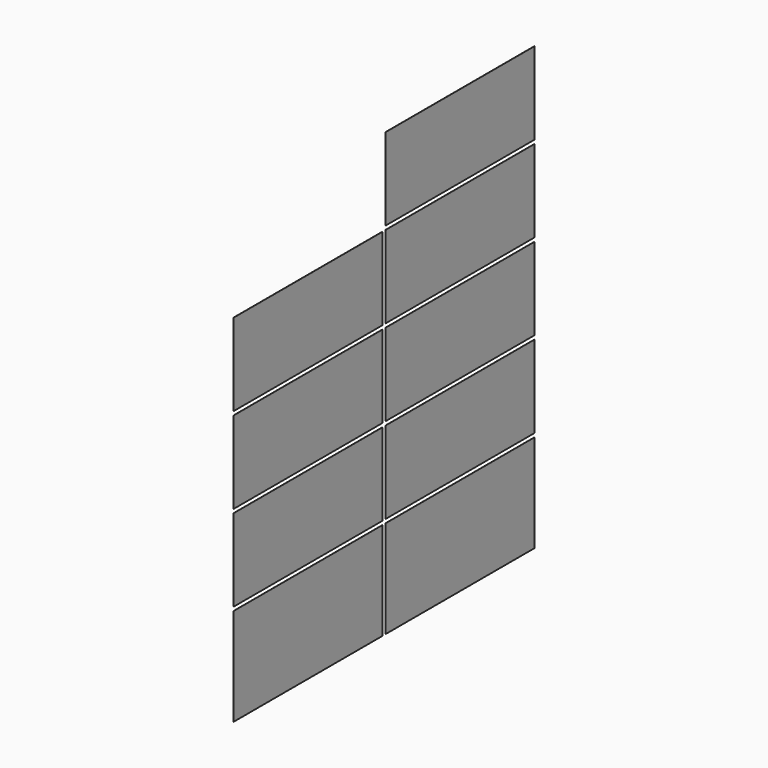
from build123d import *

# Parameters (mm, degrees)
F1_DEPTH = 0.012


# Not quite as in the source:
# - a feature names something its author has since deleted; it is built from what else it names


with BuildPart() as f1:
    # F0 (on Right) → F1 (new body)
    with BuildSketch(Plane.YZ):
        Polygon((50, -12.238), (50, -1.304), (25.25, -1.304), (25.25, -3.119), (25.25, -6.119), (25.25, -6.521), (25.25, -7.021), (25.25, -9.119), (25.25, -12.238), align=None)
    extrude(amount=F1_DEPTH)


with BuildPart() as f1b:
    # F0 (on Right) → F1, piece 2 (new body)
    with BuildSketch(Plane.YZ):
        Polygon((12.375, -12.738), (7.3750000447, -12.738), (0, -12.738), (0, -23.672), (24.75, -23.672), (24.75, -21.205), (24.75, -18.205), (24.75, -15.205), (24.75, -12.738), (17.375, -12.738), align=None)
    extrude(amount=F1_DEPTH)


with BuildPart() as f1c:
    # F0 (on Right) → F1, piece 3 (new body)
    with BuildSketch(Plane.YZ):
        Polygon((25.25, -12.738), (25.25, -15.205), (25.25, -17.955), (25.25, -18.205), (25.25, -18.455), (25.25, -21.205), (25.25, -23.672), (50, -23.672), (50, -12.738), align=None)
    extrude(amount=F1_DEPTH)


with BuildPart() as f1d:
    # F0 (on Right) → F1, piece 4 (new body)
    with BuildSketch(Plane.YZ):
        Polygon((50, -24.172), (25.25, -24.172), (25.25, -29.389), (25.25, -29.889), (25.25, -35.106), (50, -35.106), align=None)
    extrude(amount=F1_DEPTH)


with BuildPart() as f1e:
    # F0 (on Right) → F1, piece 5 (new body)
    with BuildSketch(Plane.YZ):
        Polygon((24.75, -24.172), (0, -24.172), (0, -35.106), (24.75, -35.106), (24.75, -29.889), (24.75, -29.389), align=None)
    extrude(amount=F1_DEPTH)


with BuildPart() as f1f:
    # F0 (on Right) → F1, piece 6 (new body)
    with BuildSketch(Plane.YZ):
        Polygon((24.75, -35.606), (0, -35.606), (0, -46.54), (24.75, -46.54), (24.75, -41.323), (24.75, -40.823), align=None)
    extrude(amount=F1_DEPTH)


with BuildPart() as f1g:
    # F0 (on Right) → F1, piece 7 (new body)
    with BuildSketch(Plane.YZ):
        Polygon((50, -35.606), (25.25, -35.606), (25.25, -40.823), (25.25, -41.323), (25.25, -46.54), (50, -46.54), align=None)
    extrude(amount=F1_DEPTH)


with BuildPart() as f1h:
    # F0 (on Right) → F1, piece 8 (new body)
    with BuildSketch(Plane.YZ):
        Polygon((25.25, -52.757), (25.25, -60), (50, -60), (50, -47.04), (25.25, -47.04), (25.25, -52.257), align=None)
    extrude(amount=F1_DEPTH)


with BuildPart() as f1i:
    # F0 (on Right) → F1, piece 9 (new body)
    with BuildSketch(Plane.YZ):
        Polygon((0, -47.04), (0, -60), (24.75, -60), (24.75, -52.757), (24.75, -52.257), (24.75, -47.04), align=None)
    extrude(amount=F1_DEPTH)


solid = Compound([f1.part, f1b.part, f1c.part, f1d.part, f1e.part, f1f.part, f1g.part, f1h.part, f1i.part])
